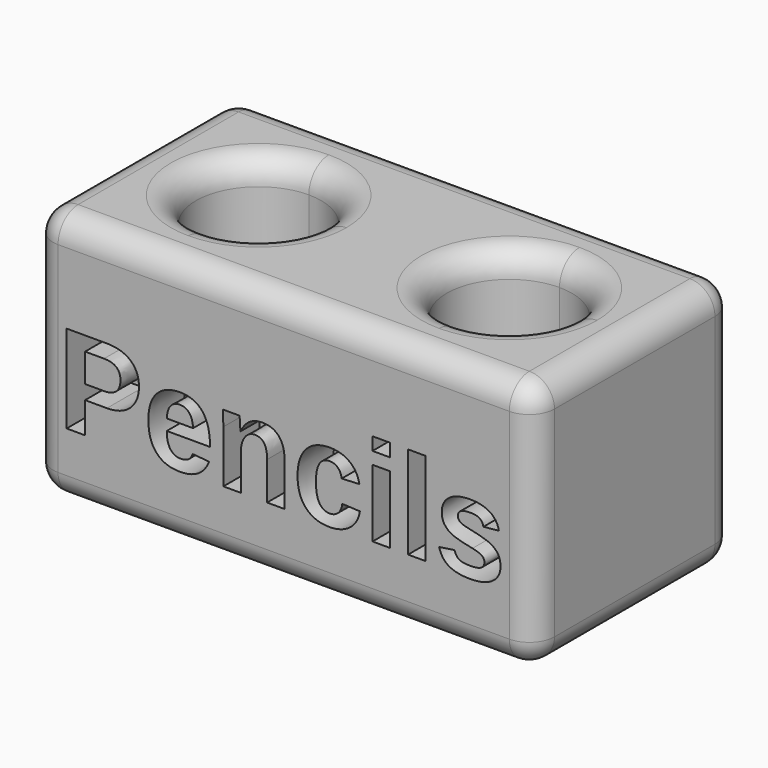
from build123d import *

# Parameters (mm, degrees)
F0_W         = 100
F0_H         = 50
F1_DEPTH     = 50
F3_DEPTH     = 60
F4_R         = 5
F5_TEXT_SIZE = 25.494622
F6_DEPTH     = 9


# Not quite as in the source:
# - Text() gives the source's letters only with a copy of the font that has no kerning and outlines rounded to 1/6400 em; it was checked with that copy


with BuildPart() as f1:
    # F0 (on Front) → F1 (new body)
    with BuildSketch(Plane.XZ):
        with Locations((0, 2.266187)):
            Rectangle(F0_W, F0_H)
    extrude(amount=F1_DEPTH)

    # F2 (on face) → F3 (cut)
    with BuildSketch(Plane.XY.offset(27.266187)):
        with BuildLine():
            ThreePointArc((-25, -12.5), (-37.5, -25), (-25, -37.5))
            Line((-25, -37.5), (-25, -12.5))
        make_face()
        with BuildLine():
            Line((-25, -12.5), (-25, -37.5))
            ThreePointArc((-25, -37.5), (-16.161165, -33.838835), (-12.5, -25))
            ThreePointArc((-12.5, -25), (-16.161165, -16.161165), (-25, -12.5))
        make_face()
        with BuildLine():
            ThreePointArc((25, -12.5), (12.5, -25), (25, -37.5))
            Line((25, -37.5), (25, -12.5))
        make_face()
        with BuildLine():
            Line((25, -12.5), (25, -37.5))
            ThreePointArc((25, -37.5), (33.838835, -33.838835), (37.5, -25))
            ThreePointArc((37.5, -25), (33.838835, -16.161165), (25, -12.5))
        make_face()
    extrude(amount=-F3_DEPTH, mode=Mode.SUBTRACT)

    # F4
    f4_edges = [f1.edges().sort_by_distance(p)[0] for p in [
        (0, -50, 27.266187),
        (-50, -25, 27.266187),
        (50, -25, 27.266187),
        (0, 0, 27.266187),
        (25, -12.5, 27.266187),
        (-50, -25, -22.733813),
        (50, -25, -22.733813),
        (-25, -12.5, 27.266187),
        (0, 0, -22.733813),
        (0, -50, -22.733813),
        (-50, -50, 2.266187),
        (50, -50, 2.266187),
        (-25, -12.5, -22.733813),
        (25, -12.5, -22.733813),
        (-50, 0, 2.266187),
        (50, 0, 2.266187),
    ]]
    fillet(f4_edges, radius=F4_R)

    # F5 (on face) → F6 (cut)
    with BuildSketch(Plane.XZ.offset(50)):
        with Locations((-45, -9.461184)):
            Text('Pencils', F5_TEXT_SIZE, font='Arimo', font_style=FontStyle.BOLD, text_align=(TextAlign.LEFT, TextAlign.BOTTOM))
    extrude(amount=-F6_DEPTH, mode=Mode.SUBTRACT)


solid = f1.part
